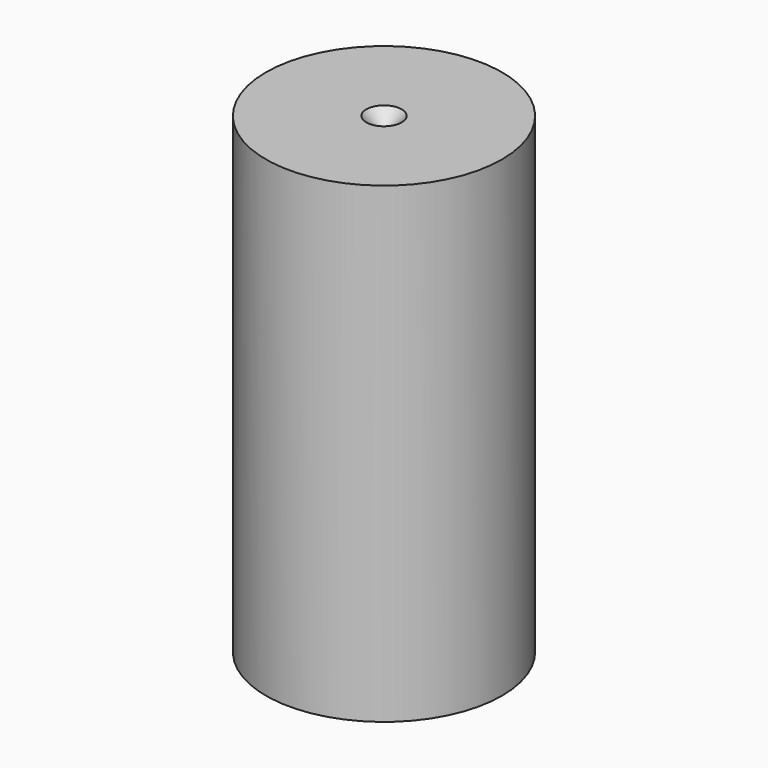
from build123d import *

# Parameters (mm, degrees)
F0_R     = 10
F1_DEPTH = 40
F2_R     = 1.5
F3_DEPTH = 1.5
F4_SIZE  = 1.49999


# Not quite as in the source:
# - a fillet or chamfer is up to 0.001 mm smaller than in the source, because OpenCascade refuses the exact size


with BuildPart() as f1:
    # F0 (on Top) → F1 (new body)
    with BuildSketch(Plane.XY):
        Circle(F0_R)
    extrude(amount=F1_DEPTH)

    # F2 (on face) → F3 (cut)
    with BuildSketch(Plane.XY.offset(40)):
        Circle(F2_R)
    extrude(amount=-F3_DEPTH, mode=Mode.SUBTRACT)

    # F4 (size 1.5 in the source; OpenCascade refuses exactly that, so slightly less here)
    f4_edges = [f1.edges().sort_by_distance(p)[0] for p in [
        (-1.5, 0, 38.5),
    ]]
    chamfer(f4_edges, length=F4_SIZE)


solid = f1.part
